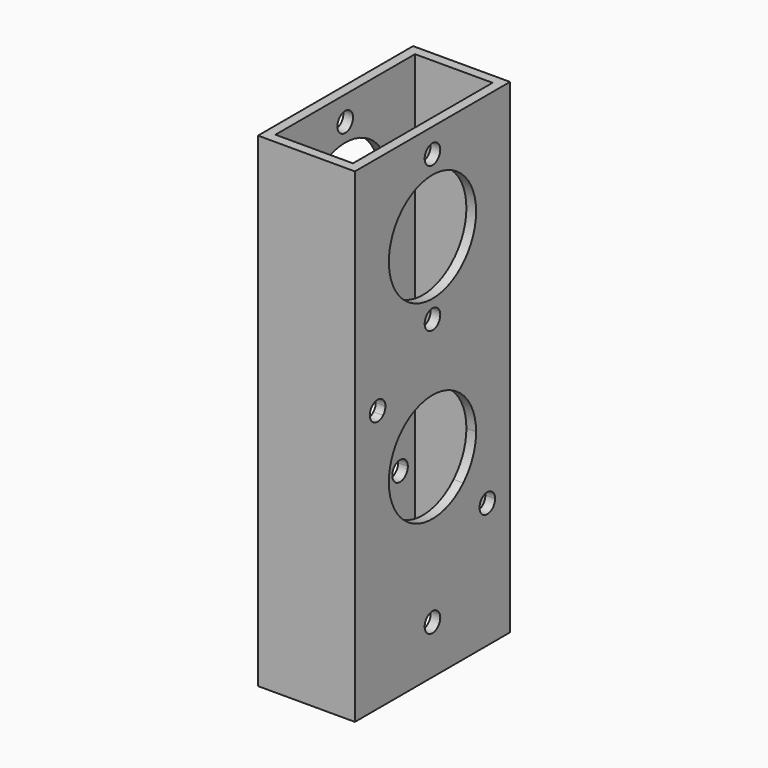
from build123d import *

# Parameters (mm, degrees)
F0_W     = 25.4
F0_H     = 50.8
F0_W_2   = 20.32
F0_H_2   = 45.72
F1_DEPTH = 127
F2_R     = 2.5527
F2_R_2   = 14.2875
F3_DEPTH = 50.8


# Not quite as in the source:
# - a feature names something its author has since deleted; it is built from what else it names


with BuildPart() as f1:
    # F0 (on Top) → F1 (new body)
    with BuildSketch(Plane.XY):
        with Locations((12.7, -25.4)):
            Rectangle(F0_W, F0_H)
        with Locations((12.7, -25.4)):
            Rectangle(F0_W_2, F0_H_2, mode=Mode.SUBTRACT)
    extrude(amount=F1_DEPTH)

    # F2 (on face) → F3 (cut)
    with BuildSketch(Plane.YZ.offset(25.4)):
        with BuildLine():
            ThreePointArc((-43.3605122421, 68.7605122421), (-42.4353064615, 69.6403379418), (-41.467058279, 70.4725605415))
            ThreePointArc((-41.467058279, 70.4725605415), (-45.1655437225, 70.5655437225), (-45.0725605415, 66.867058279))
            ThreePointArc((-45.0725605415, 66.867058279), (-44.2403379418, 67.8353064615), (-43.3605122421, 68.7605122421))
        make_face()
        with Locations((-25.4, 82.55)):
            Circle(F2_R)
        with Locations((-25.4, 12.7)):
            Circle(F2_R)
        with BuildLine():
            Line((-25.4, 50.8), (-15.2972118638, 40.6972118638))
            ThreePointArc((-15.2972118638, 40.6972118638), (-12.2000711792, 45.3324104601), (-11.1125, 50.8))
            ThreePointArc((-11.1125, 50.8), (-19.9324104601, 63.9999288208), (-35.5027881362, 60.9027881362))
            Line((-35.5027881362, 60.9027881362), (-25.4, 50.8))
        make_face()
        with BuildLine():
            Line((-25.4, 50.8), (-35.5027881362, 60.9027881362))
            ThreePointArc((-35.5027881362, 60.9027881362), (-38.5999288208, 56.2675895399), (-39.6875, 50.8))
            Line((-39.6875, 50.8), (-25.4, 50.8))
        make_face()
        with BuildLine():
            Line((-41.5554807618, 66.9554807618), (-43.3605122421, 68.7605122421))
            ThreePointArc((-43.3605122421, 68.7605122421), (-44.2403379418, 67.8353064615), (-45.0725605415, 66.867058279))
            ThreePointArc((-45.0725605415, 66.867058279), (-43.2963553886, 66.2086185946), (-41.5554807618, 66.9554807618))
        make_face()
        with BuildLine():
            ThreePointArc((-40.8078122421, 68.7605122421), (-40.9783181672, 69.6778064584), (-41.467058279, 70.4725605415))
            ThreePointArc((-41.467058279, 70.4725605415), (-42.4353064615, 69.6403379418), (-43.3605122421, 68.7605122421))
            Line((-43.3605122421, 68.7605122421), (-41.5554807618, 66.9554807618))
            ThreePointArc((-41.5554807618, 66.9554807618), (-41.0021249595, 67.7836362443), (-40.8078122421, 68.7605122421))
        make_face()
        with BuildLine():
            ThreePointArc((-39.6875, 50.8), (-30.8675895399, 37.6000711792), (-15.2972118638, 40.6972118638))
            Line((-15.2972118638, 40.6972118638), (-25.4, 50.8))
            Line((-25.4, 50.8), (-39.6875, 50.8))
        make_face()
        with BuildLine():
            ThreePointArc((-4.8867877579, 32.8394877579), (-5.1063972127, 33.8753283817), (-5.7274394585, 34.732941721))
            ThreePointArc((-5.7274394585, 34.732941721), (-6.5596620582, 33.7646935385), (-7.4394877579, 32.8394877579))
            ThreePointArc((-7.4394877579, 32.8394877579), (-8.3646935385, 31.9596620582), (-9.332941721, 31.1274394585))
            ThreePointArc((-9.332941721, 31.1274394585), (-6.5221935416, 30.4572936829), (-4.8867877579, 32.8394877579))
        make_face()
        with BuildLine():
            ThreePointArc((-7.4394877579, 32.8394877579), (-6.5596620582, 33.7646935385), (-5.7274394585, 34.732941721))
            ThreePointArc((-5.7274394585, 34.732941721), (-7.5036446114, 35.3913814054), (-9.2445192382, 34.6445192382))
            Line((-9.2445192382, 34.6445192382), (-7.4394877579, 32.8394877579))
        make_face()
        with BuildLine():
            ThreePointArc((-9.332941721, 31.1274394585), (-8.3646935385, 31.9596620582), (-7.4394877579, 32.8394877579))
            Line((-7.4394877579, 32.8394877579), (-9.2445192382, 34.6445192382))
            ThreePointArc((-9.2445192382, 34.6445192382), (-9.9913814054, 32.9036446114), (-9.332941721, 31.1274394585))
        make_face()
        with Locations((-25.4, 120.65)):
            Circle(F2_R)
        with Locations((-25.4, 101.6)):
            Circle(F2_R_2)
    extrude(amount=-F3_DEPTH, mode=Mode.SUBTRACT)


solid = f1.part
